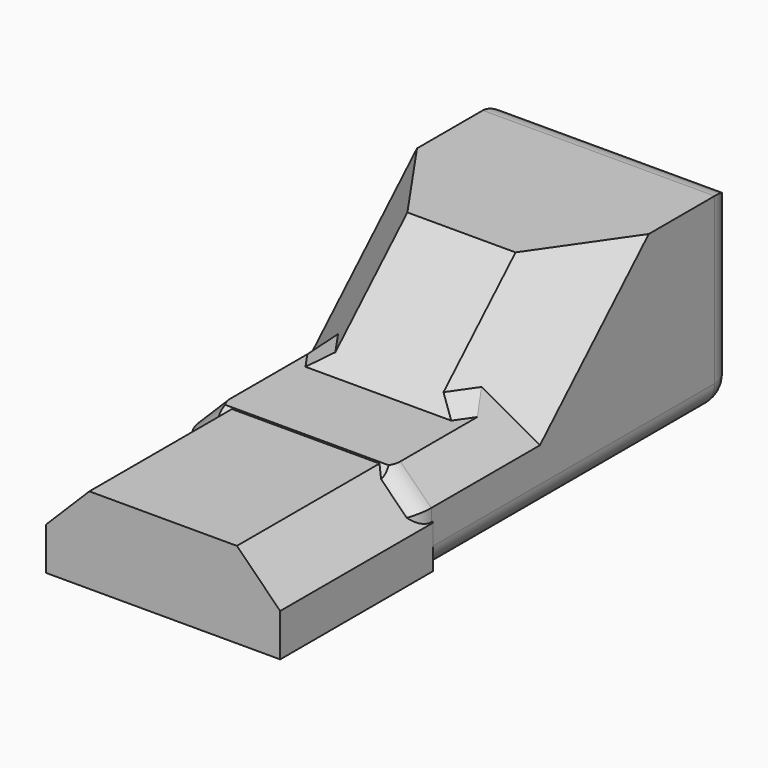
from build123d import *

# Parameters (mm, degrees)
F1_DEPTH      = 76.2
F2_SIZE       = 20.32
F3_SIZE       = 10.16
F4_SIZE       = 5.08
F5_SIZE       = 5.08
F6_SIZE       = 5.08
F7_T1_DEPTH   = 50.1089220358
F7_T3_DEPTH   = 83.82
F7_T5_DEPTH   = 32.7781013128
F7_T7_DEPTH   = 50.1089220358
F7_T9_DEPTH   = 59.0301131444
F7_T11_DEPTH  = 116.4331532733
F7_T13_DEPTH  = 119.124717139
F7_T15_DEPTH  = 75.7315738338
F7_S19_W      = 8.5849434278
F7_S19_H      = 8.5849434278
F7_T20_DEPTH  = 8.5849434278
F7_S25_W      = 8.5849434278
F7_S25_H      = 8.5849434278
F7_T26_DEPTH  = 8.5849434278
F7_S31_W      = 8.5849434278
F7_S31_H      = 8.5849434278
F7_T32_DEPTH  = 8.5849434278
F7_S37_W      = 8.5849434278
F7_S37_H      = 8.5849434278
F7_T38_DEPTH  = 8.5849434278
F8_W          = 62.888501212
F8_H          = 28.2388273627
F9_DEPTH      = 76.454
F9_DEPTH_BACK = 0.508
F10_SIZE      = 14.224


# Not quite as in the source:
# - a fillet or chamfer that OpenCascade refuses, or shapes differently, is made with other operations: its cross-section is extruded or revolved along the edge and cut away or added


with BuildPart() as f1:
    # F0 (on Right) → F1 (new body)
    with BuildSketch(Plane.YZ):
        Polygon((0, -25.0505693257), (-34.4635136425, -25.0505693257), (-34.4635136425, -55.1112554967), (99.1395264864, -55.1112554967), (99.1395264864, 7.7429031953), (34.1598689556, 7.7429031953), align=None)
    extrude(amount=F1_DEPTH)

    # F2
    f2_edges = [f1.edges().sort_by_distance(p)[0] for p in [
        (76.2, 17.079934, -8.653833),
        (0, 17.079934, -8.653833),
    ]]
    chamfer(f2_edges, length=F2_SIZE)

    # F3
    f3_edges = [f1.edges().sort_by_distance(p)[0] for p in [
        (76.2, -17.231757, -25.050569),
        (0, -17.231757, -25.050569),
    ]]
    chamfer(f3_edges, length=F3_SIZE)

    # F4
    f4_edges = [f1.edges().sort_by_distance(p)[0] for p in [
        (60.96, 7.335403, -25.050569),
    ]]
    chamfer(f4_edges, length=F4_SIZE)

    # F5
    f5_edges = [f1.edges().sort_by_distance(p)[0] for p in [
        (15.24, 7.335403, -25.050569),
    ]]
    chamfer(f5_edges, length=F5_SIZE)

    # F6
    f6_edges = [f1.edges().sort_by_distance(p)[0] for p in [
        (38.1, -34.463514, -25.050569),
    ]]
    chamfer(f6_edges, length=F6_SIZE)

    # F7: fillet of radius 8.5849434278 on 12 edges, made by hand

    # F7_s2 → F7_t1 (cut)
    with BuildSketch(Plane(origin=(2.6508946219, 0, 2.6508946219), x_dir=(0, 1, 0), z_dir=(-0.7071067812, 0, -0.7071067812))):
        with BuildLine():
            ThreePointArc((-25.8785702148, 24.8976323396), (-31.9490419287, 27.4121040535), (-34.4635136425, 33.4825757674))
            Line((-34.4635136425, 33.4825757674), (-34.4635136425, 24.8976323396))
            Line((-34.4635136425, 24.8976323396), (-25.8785702148, 24.8976323396))
        make_face()
    extrude(amount=F7_T1_DEPTH, mode=Mode.SUBTRACT)

    # F7_s4 → F7_t3 (cut)
    with BuildSketch(Plane.YZ.offset(-3.81)):
        with BuildLine():
            ThreePointArc((-31.9490419287, -27.6160976118), (-33.8100237355, -30.4012537081), (-34.4635136425, -33.6865693257))
            Line((-34.4635136425, -33.6865693257), (-34.4635136425, -30.1305693257))
            Line((-34.4635136425, -30.1305693257), (-31.9490419287, -27.6160976118))
        make_face()
    extrude(amount=F7_T3_DEPTH, mode=Mode.SUBTRACT)

    # F7_s6 → F7_t5 (cut)
    with BuildSketch(Plane.XY.offset(-46.5263120689)):
        with BuildLine():
            ThreePointArc((8.5849434278, -34.4635136425), (2.5144717139, -31.9490419287), (0, -25.8785702148))
            Line((0, -25.8785702148), (0, -34.4635136425))
            Line((0, -34.4635136425), (8.5849434278, -34.4635136425))
        make_face()
        with BuildLine():
            ThreePointArc((67.6150565722, -34.4635136425), (73.6855282861, -31.9490419287), (76.2, -25.8785702148))
            Line((76.2, -25.8785702148), (76.2, -34.4635136425))
            Line((76.2, -34.4635136425), (67.6150565722, -34.4635136425))
        make_face()
    extrude(amount=F7_T5_DEPTH, mode=Mode.SUBTRACT)

    # F7_s8 → F7_t7 (cut)
    with BuildSketch(Plane(origin=(35.4491053781, 0, -35.4491053781), x_dir=(0, 1, 0), z_dir=(0.7071067812, 0, -0.7071067812))):
        with BuildLine():
            ThreePointArc((-25.8785702148, 28.9839043868), (-31.9490419287, 26.4694326729), (-34.4635136425, 20.398960959))
            Line((-34.4635136425, 20.398960959), (-34.4635136425, 28.9839043868))
            Line((-34.4635136425, 28.9839043868), (-25.8785702148, 28.9839043868))
        make_face()
    extrude(amount=F7_T7_DEPTH, mode=Mode.SUBTRACT)

    # F7_s10 → F7_t9 (cut)
    with BuildSketch(Plane.YZ.offset(8.5849434278)):
        with BuildLine():
            ThreePointArc((-34.4635136425, -46.5263120689), (-31.9490419287, -52.5967837828), (-25.8785702148, -55.1112554967))
            Line((-25.8785702148, -55.1112554967), (-34.4635136425, -55.1112554967))
            Line((-34.4635136425, -55.1112554967), (-34.4635136425, -46.5263120689))
        make_face()
        with BuildLine():
            ThreePointArc((90.5545830586, -55.1112554967), (96.6250547725, -52.5967837828), (99.1395264864, -46.5263120689))
            Line((99.1395264864, -46.5263120689), (99.1395264864, -55.1112554967))
            Line((99.1395264864, -55.1112554967), (90.5545830586, -55.1112554967))
        make_face()
    extrude(amount=F7_T9_DEPTH, mode=Mode.SUBTRACT)

    # F7_s12 → F7_t11 (cut)
    with BuildSketch(Plane.XZ.offset(-90.5545830586)):
        with BuildLine():
            ThreePointArc((0, -46.5263120689), (2.5144717139, -52.5967837828), (8.5849434278, -55.1112554967))
            Line((8.5849434278, -55.1112554967), (0, -55.1112554967))
            Line((0, -55.1112554967), (0, -46.5263120689))
        make_face()
        with BuildLine():
            ThreePointArc((76.2, -46.5263120689), (73.6855282861, -52.5967837828), (67.6150565722, -55.1112554967))
            Line((67.6150565722, -55.1112554967), (76.2, -55.1112554967))
            Line((76.2, -55.1112554967), (76.2, -46.5263120689))
        make_face()
    extrude(amount=F7_T11_DEPTH, mode=Mode.SUBTRACT)

    # F7_s14 → F7_t13 (cut)
    with BuildSketch(Plane.YZ.offset(-21.4623585695)):
        with BuildLine():
            ThreePointArc((90.5545830586, 7.7429031953), (96.6250547725, 5.2284314814), (99.1395264864, -0.8420402325))
            Line((99.1395264864, -0.8420402325), (99.1395264864, 7.7429031953))
            Line((99.1395264864, 7.7429031953), (90.5545830586, 7.7429031953))
        make_face()
    extrude(amount=F7_T13_DEPTH, mode=Mode.SUBTRACT)

    # F7_s16 → F7_t15 (cut)
    with BuildSketch(Plane.XY.offset(-46.5263120689)):
        with BuildLine():
            ThreePointArc((0, 90.5545830586), (2.5144717139, 96.6250547725), (8.5849434278, 99.1395264864))
            Line((8.5849434278, 99.1395264864), (0, 99.1395264864))
            Line((0, 99.1395264864), (0, 90.5545830586))
        make_face()
        with BuildLine():
            ThreePointArc((76.2, 90.5545830586), (73.6855282861, 96.6250547725), (67.6150565722, 99.1395264864))
            Line((67.6150565722, 99.1395264864), (76.2, 99.1395264864))
            Line((76.2, 99.1395264864), (76.2, 90.5545830586))
        make_face()
    extrude(amount=F7_T15_DEPTH, mode=Mode.SUBTRACT)


with BuildPart() as f7_tool18:
    # F7_s19 → F7_t20 (new body)
    with BuildSketch(Plane.XZ.offset(25.8785702148)):
        with Locations((4.2924717139, -50.8187837828)):
            Rectangle(F7_S19_W, F7_S19_H)
    extrude(amount=F7_T20_DEPTH)

    # F7_s21 → F7_t22 (revolve, cut)
    with BuildSketch(Plane(origin=(8.5849434278, -25.8785702148, -46.5263120689), x_dir=(0.7071067812, 0, 0.7071067812), z_dir=(0.7071067812, 0, -0.7071067812))):
        with BuildLine():
            ThreePointArc((0, -8.5849434278), (8.5849434278, 0), (0, 8.5849434278))
            Line((0, 8.5849434278), (0, -8.5849434278))
        make_face()
    revolve(axis=Axis((8.5849434278, -25.8785702148, -46.5263120689), (0, -1, 0)), mode=Mode.SUBTRACT)


with BuildPart() as f1_1:
    add(f1.part)

    # F7_t17: cut F7_tool18
    add(f7_tool18.part, mode=Mode.SUBTRACT)


with BuildPart() as f7_tool24:
    # F7_s25 → F7_t26 (new body)
    with BuildSketch(Plane.XZ.offset(25.8785702148)):
        with Locations((71.9075282861, -50.8187837828)):
            Rectangle(F7_S25_W, F7_S25_H)
    extrude(amount=F7_T26_DEPTH)

    # F7_s27 → F7_t28 (revolve, cut)
    with BuildSketch(Plane(origin=(67.6150565722, -25.8785702148, -46.5263120689), x_dir=(-0.7071067812, 0, 0.7071067812), z_dir=(0.7071067812, 0, 0.7071067812))):
        with BuildLine():
            ThreePointArc((0, -8.5849434278), (8.5849434278, 0), (0, 8.5849434278))
            Line((0, 8.5849434278), (0, -8.5849434278))
        make_face()
    revolve(axis=Axis((67.6150565722, -25.8785702148, -46.5263120689), (0, -1, 0)), mode=Mode.SUBTRACT)


with BuildPart() as f1_2:
    add(f1_1.part)

    # F7_t23: cut F7_tool24
    add(f7_tool24.part, mode=Mode.SUBTRACT)


with BuildPart() as f7_tool30:
    # F7_s31 → F7_t32 (new body)
    with BuildSketch(Plane.XZ.offset(-90.5545830586)):
        with Locations((4.2924717139, -50.8187837828)):
            Rectangle(F7_S31_W, F7_S31_H)
    extrude(amount=-F7_T32_DEPTH)

    # F7_s33 → F7_t34 (revolve, cut)
    with BuildSketch(Plane(origin=(8.5849434278, 90.5545830586, -46.5263120689), x_dir=(0.7071067812, 0, 0.7071067812), z_dir=(-0.7071067812, 0, 0.7071067812))):
        with BuildLine():
            ThreePointArc((0, -8.5849434278), (8.5849434278, 0), (0, 8.5849434278))
            Line((0, 8.5849434278), (0, -8.5849434278))
        make_face()
    revolve(axis=Axis((8.5849434278, 90.5545830586, -46.5263120689), (0, 1, 0)), mode=Mode.SUBTRACT)


with BuildPart() as f1_3:
    add(f1_2.part)

    # F7_t29: cut F7_tool30
    add(f7_tool30.part, mode=Mode.SUBTRACT)


with BuildPart() as f7_tool36:
    # F7_s37 → F7_t38 (new body)
    with BuildSketch(Plane.XZ.offset(-90.5545830586)):
        with Locations((71.9075282861, -50.8187837828)):
            Rectangle(F7_S37_W, F7_S37_H)
    extrude(amount=-F7_T38_DEPTH)

    # F7_s39 → F7_t40 (revolve, cut)
    with BuildSketch(Plane(origin=(67.6150565722, 90.5545830586, -46.5263120689), x_dir=(-0.7071067812, 0, 0.7071067812), z_dir=(-0.7071067812, 0, -0.7071067812))):
        with BuildLine():
            ThreePointArc((0, -8.5849434278), (8.5849434278, 0), (0, 8.5849434278))
            Line((0, 8.5849434278), (0, -8.5849434278))
        make_face()
    revolve(axis=Axis((67.6150565722, 90.5545830586, -46.5263120689), (0, 1, 0)), mode=Mode.SUBTRACT)


with BuildPart() as f1_4:
    add(f1_3.part)

    # F7_t35: cut F7_tool36
    add(f7_tool36.part, mode=Mode.SUBTRACT)


with BuildPart() as f9:
    # F8 (on Right) → F9 (new body, two sides)
    with BuildSketch(Plane.YZ) as f9_sk:
        with Locations((-56.8328062072, -39.4736258313)):
            Rectangle(F8_W, F8_H)
    extrude(amount=F9_DEPTH)
    extrude(f9_sk.sketch, amount=-F9_DEPTH_BACK)

    # F10
    f10_edges = [f9.edges().sort_by_distance(p)[0] for p in [
        (76.454, -56.832806, -25.354212),
        (-0.508, -56.832806, -25.354212),
    ]]
    chamfer(f10_edges, length=F10_SIZE)


solid = Compound([f1_4.part, f9.part])
